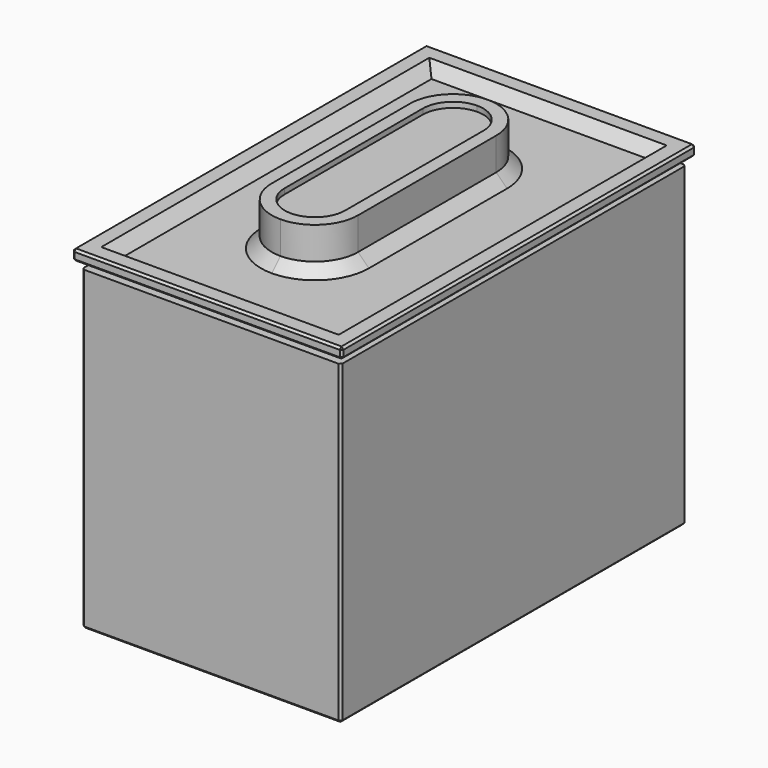
from build123d import *

# Parameters (mm, degrees)
F0_W      = 12
F0_H      = 15
F1_DEPTH  = 20
F3_DEPTH  = 1
F4_W      = 12.5
F4_H      = 20.5
F4_W_2    = 12
F4_H_2    = 20
F5_DEPTH  = 0.5
F7_DEPTH  = 0.5
F9_DEPTH  = 2
F10_DEPTH = 1.75
F11_SIZE  = 0.1
F12_SIZE  = 0.49999
F13_W     = 2.4198924027
F13_H     = 0.5
F13_W_2   = 11.8
F13_W_3   = 1.8122543529
F14_DEPTH = 25
F15_DEPTH = 0.25


# Not quite as in the source:
# - a fillet or chamfer is up to 0.001 mm smaller than in the source, because OpenCascade refuses the exact size


with BuildPart() as f1:
    # F0 (on Front) → F1 (new body)
    with BuildSketch(Plane.XZ):
        with Locations((6, 7.5)):
            Rectangle(F0_W, F0_H)
    extrude(amount=F1_DEPTH)

    # F2 (on face) → F3 (join)
    with BuildSketch(Plane(origin=(0, 0, 0), x_dir=(0, -1, 0), z_dir=(-1, 0, 0))):
        with BuildLine():
            ThreePointArc((10.5, 7.5), (10.158113883, 7.974341649), (9.6, 7.8))
            Line((9.6, 7.8), (10.4, 7.2))
            ThreePointArc((10.4, 7.2), (10.474341649, 7.341886117), (10.5, 7.5))
        make_face()
        with BuildLine():
            Line((10.4, 7.2), (9.6, 7.8))
            ThreePointArc((9.6, 7.8), (9.7, 7.1), (10.4, 7.2))
        make_face()
    extrude(amount=F3_DEPTH)

    # F4 (on face) → F5 (join)
    with BuildSketch(Plane.XY.offset(15)):
        with Locations((6, -10)):
            Rectangle(F4_W, F4_H)
        with Locations((6, -10)):
            Rectangle(F4_W_2, F4_H_2, mode=Mode.SUBTRACT)
        Polygon((12, 0), (0, 0), (12, -20), align=None)
        Polygon((12, -20), (0, 0), (0, -20), align=None)
    extrude(amount=F5_DEPTH)

    # F6 (on face) → F7 (cut)
    with BuildSketch(Plane.XY.offset(15.5)):
        Polygon((11.5, -19.02), (0.5, -0.98), (0.5, -19.5), (11.5, -19.5), align=None)
        Polygon((0.5, -0.5), (0.5, -0.98), (11.5, -19.02), (11.5, -0.5), align=None)
    extrude(amount=-F7_DEPTH, mode=Mode.SUBTRACT)

    # F8 (on face) → F9 (join)
    with BuildSketch(Plane.XY.offset(15)):
        Polygon((4.6, -7.5818181818), (4, -6.5454545455), (4, -14), (4.6, -14), align=None)
        Polygon((4, -6), (4, -6.5454545455), (4.6, -7.5818181818), (4.6, -6), align=None)
        with BuildLine():
            ThreePointArc((6, -4), (4.5857864376, -4.5857864376), (4, -6))
            Line((4, -6), (4.6, -6))
            Line((4.6, -6), (4.6, -4.6))
            Line((4.6, -4.6), (6, -4.6))
            Line((6, -4.6), (7.4, -4.6))
            Line((7.4, -4.6), (7.4, -6))
            Line((7.4, -6), (8, -6))
            ThreePointArc((8, -6), (7.4142135624, -4.5857864376), (6, -4))
        make_face()
        with BuildLine():
            Line((4.6, -4.6), (4.6, -6))
            ThreePointArc((4.6, -6), (5.0100505063, -5.0100505063), (6, -4.6))
            Line((6, -4.6), (4.6, -4.6))
        make_face()
        with BuildLine():
            ThreePointArc((6, -4.6), (6.9899494937, -5.0100505063), (7.4, -6))
            Line((7.4, -6), (7.4, -4.6))
            Line((7.4, -4.6), (6, -4.6))
        make_face()
        Polygon((7.4, -6), (7.4, -12.4181818182), (8, -13.4545454545), (8, -6), align=None)
        Polygon((8, -13.4545454545), (7.4, -12.4181818182), (7.4, -14), (8, -14), align=None)
        with BuildLine():
            Line((4.6, -14), (4, -14))
            ThreePointArc((4, -14), (4.5857864376, -15.4142135624), (6, -16))
            ThreePointArc((6, -16), (7.4142135624, -15.4142135624), (8, -14))
            Line((8, -14), (7.4, -14))
            Line((7.4, -14), (7.4, -15.4))
            Line((7.4, -15.4), (6, -15.4))
            Line((6, -15.4), (4.6, -15.4))
            Line((4.6, -15.4), (4.6, -14))
        make_face()
        with BuildLine():
            Line((7.4, -15.4), (7.4, -14))
            ThreePointArc((7.4, -14), (6.9899494937, -14.9899494937), (6, -15.4))
            Line((6, -15.4), (7.4, -15.4))
        make_face()
        with BuildLine():
            ThreePointArc((6, -15.4), (5.0100505063, -14.9899494937), (4.6, -14))
            Line((4.6, -14), (4.6, -15.4))
            Line((4.6, -15.4), (6, -15.4))
        make_face()
    extrude(amount=F9_DEPTH)

    # F10 (add): a face of the model
    f10_faces = [f1.faces().sort_by_distance(p)[0] for p in [
        (6, -10, 15),
    ]]
    extrude(f10_faces, amount=F10_DEPTH)

    # F11
    f11_edges = [f1.edges().sort_by_distance(p)[0] for p in [
        (0, 0, 7.5),
        (0, -10, 0),
        (6, 0, 0),
        (0, -20, 7.5),
        (6, -20, 0),
        (12, -20, 7.5),
        (12, 0, 7.5),
        (12, -10, 0),
        (12.25, -20.25, 15.25),
        (12.25, 0.25, 15.25),
        (12.25, -10, 15),
        (12, -10, 15),
        (6, -20, 15),
        (6, -20.25, 15),
        (0, -10, 15),
        (-0.25, -20.25, 15.25),
        (-0.25, -10, 15),
        (6, 0.25, 15),
        (-0.25, 0.25, 15.25),
        (6, 0.25, 15.5),
        (-0.25, -10, 15.5),
        (12.25, -10, 15.5),
        (6, -20.25, 15.5),
        (6, 0, 15),
    ]]
    chamfer(f11_edges, length=F11_SIZE)

    # F12 (size 0.5 in the source; OpenCascade refuses exactly that, so slightly less here)
    f12_edges = [f1.edges().sort_by_distance(p)[0] for p in [
        (0.5, -10, 15),
        (6, -0.5, 15),
        (11.5, -10, 15),
        (6, -19.5, 15),
        (8, -10, 15),
        (6, -4, 15),
        (4, -10, 15),
        (6, -16, 15),
    ]]
    chamfer(f12_edges, length=F12_SIZE)

    # F13 (on face) → F14 (cut)
    with BuildSketch(Plane.XZ.offset(20)):
        with Locations((-1.1099462014, 14.65)):
            Rectangle(F13_W, F13_H)
        with Locations((6, 14.65)):
            Rectangle(F13_W_2, F13_H)
        with Locations((12.8061271764, 14.65)):
            Rectangle(F13_W_3, F13_H)
    extrude(amount=-F14_DEPTH, mode=Mode.SUBTRACT)

    # F15 (add): a face of the model
    f15_faces = [f1.faces().sort_by_distance(p)[0] for p in [
        (6, -10, 14.4),
    ]]
    extrude(f15_faces, amount=F15_DEPTH)


solid = f1.part
